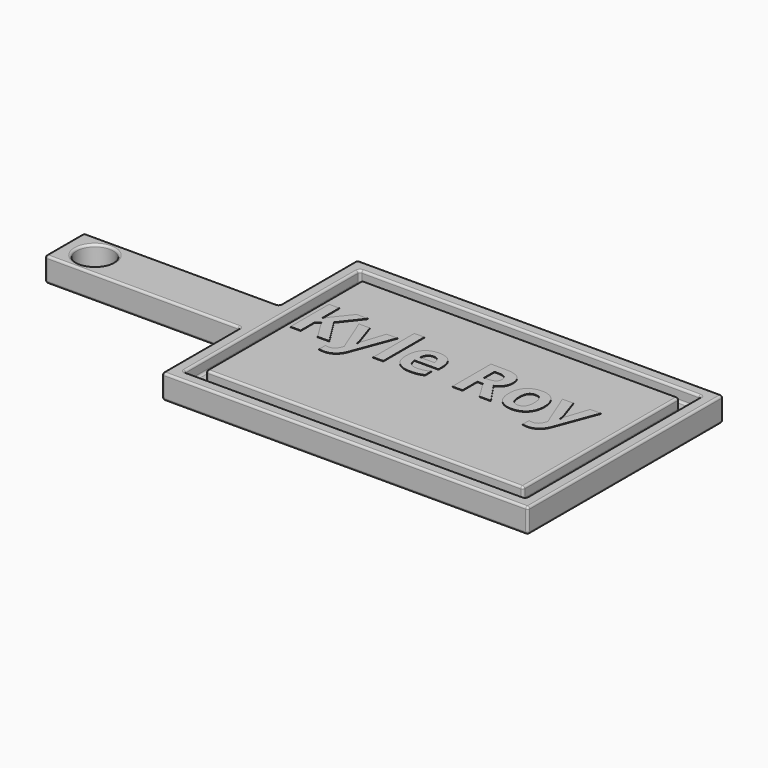
from build123d import *

# Parameters (mm, degrees)
F0_W         = 203.2
F0_H         = 50.8
F1_DEPTH     = 25.4
F2_R         = 19.05
F3_DEPTH     = 25.4
F5_DEPTH     = 12.7
F6_R         = 2.286
F7_TEXT_SIZE = 70.5555555556
F8_DEPTH     = 0.508


# Not quite as in the source:
# - Text() gives the source's letters only with a copy of the font that has no kerning and outlines rounded to 1/6400 em; it was checked with that copy


with BuildPart() as f1:
    # F0 (on Top) → F1 (new body)
    with BuildSketch(Plane.XY):
        Polygon((0, 101.6), (0, 0), (381, 0), (381, 254), (0, 254), (0, 152.4), align=None)
        with Locations((-101.6, 127)):
            Rectangle(F0_W, F0_H)
    extrude(amount=F1_DEPTH)

    # F2 (on face) → F3 (cut)
    with BuildSketch(Plane.XY.offset(25.4)):
        with Locations((-171.45, 127)):
            Circle(F2_R)
    extrude(amount=-F3_DEPTH, mode=Mode.SUBTRACT)

    # F4 (on face) → F5 (cut)
    with BuildSketch(Plane.XY.offset(25.4)):
        Polygon((12.7, 101.6), (12.7, 12.7), (368.3, 12.7), (368.3, 241.3), (12.7, 241.3), (12.7, 152.4), align=None)
        Polygon((25.4000046253, 101.6), (25.4000046253, 152.4), (25.4000046253, 228.5999953747), (355.5999953747, 228.5999953747), (355.5999953747, 25.4000046253), (25.4000046253, 25.4000046253), align=None, mode=Mode.SUBTRACT)
    extrude(amount=-F5_DEPTH, mode=Mode.SUBTRACT)

    # F6
    f6_edges = [f1.edges().sort_by_distance(p)[0] for p in [
        (-203.2, 101.6, 12.7),
        (0, 101.6, 12.7),
        (-101.6, 101.6, 0),
        (-101.6, 101.6, 25.4),
        (-203.2, 152.4, 12.7),
        (-203.2, 127, 0),
        (-203.2, 127, 25.4),
        (0, 152.4, 12.7),
        (-101.6, 152.4, 0),
        (-101.6, 152.4, 25.4),
        (0, 254, 12.7),
        (0, 203.2, 0),
        (0, 203.2, 25.4),
        (0, 0, 12.7),
        (0, 50.8, 0),
        (0, 50.8, 25.4),
        (381, 0, 12.7),
        (190.5, 0, 0),
        (190.5, 0, 25.4),
        (381, 254, 12.7),
        (381, 127, 0),
        (381, 127, 25.4),
        (190.5, 254, 0),
        (190.5, 254, 25.4),
        (25.400005, 228.599995, 19.05),
        (355.599995, 228.599995, 19.05),
        (190.5, 228.599995, 25.4),
        (190.5, 228.599995, 12.7),
        (-190.5, 127, 25.4),
        (190.5, 12.7, 25.4),
        (368.3, 127, 25.4),
        (190.5, 241.3, 25.4),
        (12.7, 127, 25.4),
        (355.599995, 25.400005, 19.05),
        (25.400005, 25.400005, 19.05),
        (190.5, 25.400005, 25.4),
        (190.5, 25.400005, 12.7),
        (355.599995, 127, 25.4),
        (25.400005, 127, 25.4),
        (25.400005, 127, 12.7),
        (368.3, 241.3, 19.05),
        (12.7, 241.3, 19.05),
        (190.5, 241.3, 12.7),
        (12.7, 12.7, 19.05),
        (12.7, 127, 12.7),
        (368.3, 12.7, 19.05),
        (368.3, 127, 12.7),
        (190.5, 12.7, 12.7),
        (355.599995, 127, 12.7),
        (-152.4, 127, 12.7),
        (-190.5, 127, 0),
    ]]
    fillet(f6_edges, radius=F6_R)

    # F7 (on face) → F8 (join)
    with BuildSketch(Plane.XY.offset(25.4)):
        with Locations((25.4513255945, 127.3783921736)):
            Text('Kyle Roy', F7_TEXT_SIZE, font='Open Sans', font_style=FontStyle.BOLD, text_align=(TextAlign.LEFT, TextAlign.BOTTOM))
    extrude(amount=F8_DEPTH)


solid = f1.part
